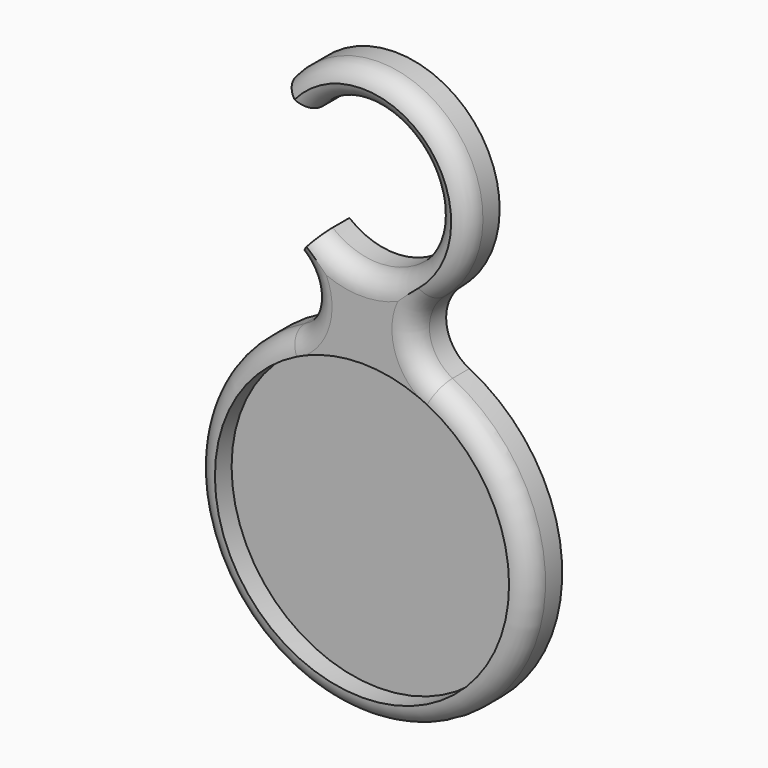
from build123d import *

# Parameters (mm, degrees)
F1_DEPTH     = 10
F2_R         = 35.25
F3_DEPTH     = 5
F4_T2_ANGLE  = 219.3901803432
F4_T4_ANGLE  = 351.1589703018
F4_T6_ANGLE  = 186.0321901893
F4_T8_ANGLE  = 307.350846925
F4_T10_ANGLE = 114.3660006612


# Not quite as in the source:
# - a fillet or chamfer that OpenCascade refuses, or shapes differently, is made with other operations: its cross-section is extruded or revolved along the edge and cut away or added


with BuildPart() as f1:
    # F0 (on Front) → F1 (new body)
    with BuildSketch(Plane.XZ):
        with BuildLine():
            ThreePointArc((-15.8377032244, 52.5521751562), (-12.2369163429, 43.6840965993), (-17.7382276114, 35.8518518519))
            ThreePointArc((-17.7382276114, 35.8518518519), (0, -40), (17.7382276114, 35.8518518519))
            ThreePointArc((17.7382276114, 35.8518518519), (12.2369163429, 43.6840965993), (15.8377032244, 52.5521751562))
            ThreePointArc((15.8377032244, 52.5521751562), (17.783880992, 89.4663920653), (-19.151111078, 87.9652662517))
            Line((-19.151111078, 87.9652662517), (-13.4057777546, 83.1443591791))
            ThreePointArc((-13.4057777546, 83.1443591791), (17.4196300213, 73.5708341746), (-11.0162958531, 58.2981047124))
            Line((-11.0162958531, 58.2981047124), (-15.8377032244, 52.5521751562))
        make_face()
    extrude(amount=F1_DEPTH)

    # F2 (on face) → F3 (cut)
    with BuildSketch(Plane.XZ.offset(10)):
        Circle(F2_R)
    extrude(amount=-F3_DEPTH, mode=Mode.SUBTRACT)

    # F4: fillet of radius 5 on 7 edges, made by hand

    # F4_s1 → F4_t2 (revolve, cut)
    with BuildSketch(Plane(origin=(35.2409155406, 0, 28.8540348163), x_dir=(0, 1, 0), z_dir=(-0.7737360341, 0, -0.633508129))):
        with BuildLine():
            ThreePointArc((-10, -35.6281978535), (-8.5355339059, -32.0926639476), (-5, -30.6281978535))
            Line((-5, -30.6281978535), (-10, -30.6281978535))
            Line((-10, -30.6281978535), (-10, -35.6281978535))
        make_face()
    revolve(axis=Axis((0, -10, 71.8955760095), (0, -1, 0)), revolution_arc=F4_T2_ANGLE, mode=Mode.SUBTRACT)

    # F4_s3 → F4_t4 (revolve, cut)
    with BuildSketch(Plane(origin=(-1.345809042, 0, 71.8703750561), x_dir=(0, 1, 0), z_dir=(0.0187222225, 0, -0.9998247238))):
        with BuildLine():
            ThreePointArc((-10, -21.1539550284), (-8.5355339059, -17.6184211225), (-5, -16.1539550284))
            Line((-5, -16.1539550284), (-10, -16.1539550284))
            Line((-10, -16.1539550284), (-10, -21.1539550284))
        make_face()
    revolve(axis=Axis((0, -10, 71.8955760095), (0, 1, 0)), revolution_arc=F4_T4_ANGLE, mode=Mode.SUBTRACT)

    # F4_s5 → F4_t6 (revolve, cut)
    with BuildSketch(Plane(origin=(4.4385257703, 0, 2.812078366), x_dir=(0, 1, 0), z_dir=(-0.8447320002, 0, -0.5351895439))):
        with BuildLine():
            ThreePointArc((-5, -59.7231505865), (-8.5355339059, -61.1876166806), (-10, -64.7231505865))
            Line((-10, -64.7231505865), (-10, -59.7231505865))
            Line((-10, -59.7231505865), (-5, -59.7231505865))
        make_face()
    revolve(axis=Axis((-22.1727845142, -10, 44.8148148148), (0, 1, 0)), revolution_arc=F4_T6_ANGLE, mode=Mode.SUBTRACT)

    # F4_s7 → F4_t8 (revolve, cut)
    with BuildSketch(Plane(origin=(0, 0, 0), x_dir=(0, 1, 0), z_dir=(0.8962962963, 0, 0.4434556903))):
        with BuildLine():
            ThreePointArc((-5, 40), (-8.5355339059, 38.5355339059), (-10, 35))
            Line((-10, 35), (-10, 40))
            Line((-10, 40), (-5, 40))
        make_face()
    revolve(axis=Axis((0, -10, 0), (0, -1, 0)), revolution_arc=F4_T8_ANGLE, mode=Mode.SUBTRACT)

    # F4_s9 → F4_t10 (revolve, cut)
    with BuildSketch(Plane(origin=(0, 0, 0), x_dir=(0, 1, 0), z_dir=(0.8962962963, 0, -0.4434556903))):
        with BuildLine():
            ThreePointArc((-10, 35), (-8.5355339059, 38.5355339059), (-5, 40))
            Line((-5, 40), (-10, 40))
            Line((-10, 40), (-10, 35))
        make_face()
    revolve(axis=Axis((22.1727845142, -10, 44.8148148148), (0, 1, 0)), revolution_arc=F4_T10_ANGLE, mode=Mode.SUBTRACT)


solid = f1.part
